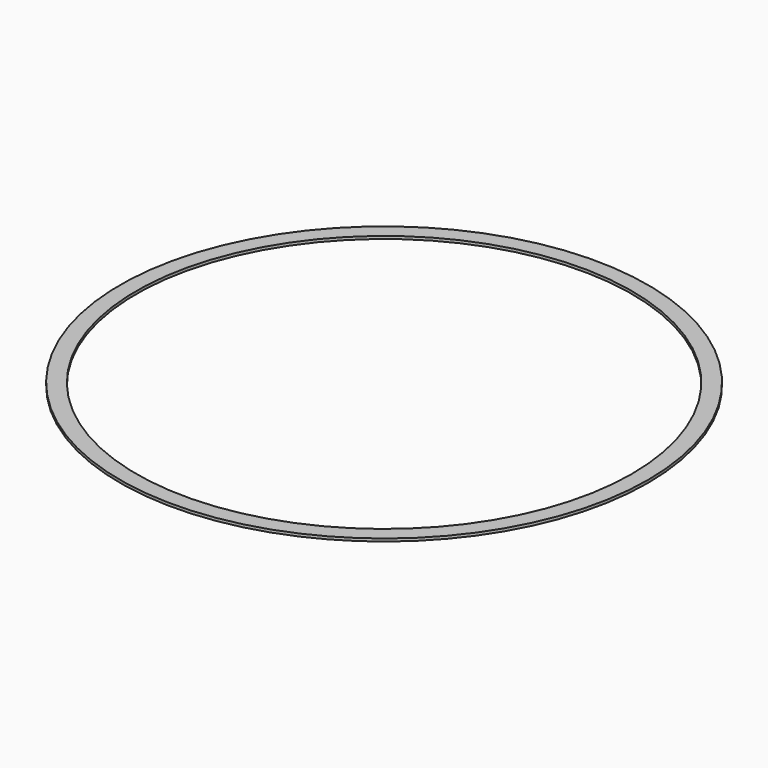
from build123d import *

# Parameters (mm, degrees)
F0_R     = 413.7406
F0_R_2   = 388.3406
F1_DEPTH = 4.2333333333


# Not quite as in the source:
# - a length typed as a fraction of an inch, garbled in the dataset ("3 / 203.2 mm" for 3/8 in), is restored


with BuildPart() as f1:
    # F0 (on Top) → F1 (new body)
    with BuildSketch(Plane.XY):
        Circle(F0_R)
        Circle(F0_R_2, mode=Mode.SUBTRACT)
    extrude(amount=F1_DEPTH)


solid = f1.part
